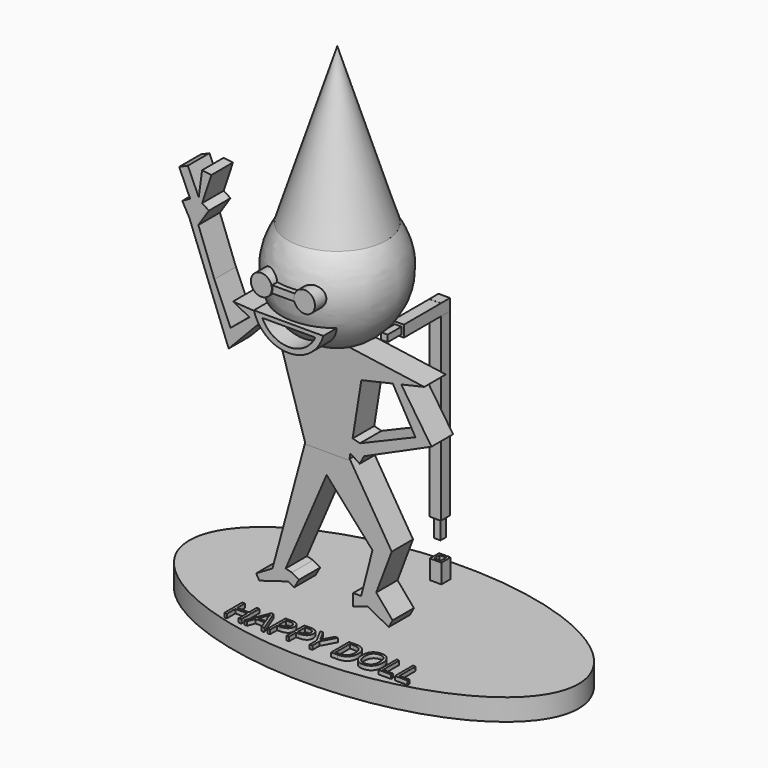
from build123d import *

# Parameters (mm, degrees)
F4_R          = 1.3944726586
F5_DEPTH      = 8.83985
F6_W          = 3.6523307208
F6_H          = 0.9525045753
F7_DEPTH      = 8.73121
F9_DEPTH      = 8.04328
F11_DEPTH     = 1.790545
F13_DEPTH     = 1.76659
F17_W         = 1.524
F17_H         = 1.524
F17_W_2       = 0.889
F17_H_2       = 0.889
F18_DEPTH     = 2.54
F21_DEPTH     = 2.87519
F23_W         = 1.524
F23_H         = 1.524
F23_W_2       = 0.889
F23_H_2       = 0.889
F24_DEPTH     = 2.54
F25_W         = 1.524
F25_H         = 1.524
F26_DEPTH     = 25.4
F28_W         = 0.889
F28_H         = 0.889
F29_DEPTH     = 2.54
F31_W         = 1.524
F31_H         = 1.524
F32_DEPTH     = 7.62
F34_W         = 0.889
F34_H         = 0.889
F35_DEPTH     = 2.286
F40_TEXT_SIZE = 4.1768032437
F41_DEPTH     = 0.52886


# Not quite as in the source:
# - a feature names something its author has since deleted; it is built from what else it names
# - Text() gives the source's letters only with a copy of the font that has no kerning and outlines rounded to 1/6400 em; it was checked with that copy


with BuildPart() as f1:
    # F0 (on Front) → F1 (revolve)
    with BuildSketch(Plane.XZ):
        with BuildLine():
            Line((0, 41.7647510767), (0, 24.1672452539))
            ThreePointArc((0, 24.1672452539), (8.0870628543, 32.9659981653), (0, 41.7647510767))
        make_face()
    revolve(axis=Axis((0, 0, 32.9659981653), (0, 0, 1)))

    # F4 (on Front) → F5 (join)
    with BuildSketch(Plane.XZ):
        with Locations((2.7146725915, 33.2950428128)):
            Circle(F4_R)
        with Locations((-3.0039404519, 33.4141813219)):
            Circle(F4_R)
    extrude(amount=F5_DEPTH)

    # F6 (on Front) → F7 (join)
    with BuildSketch(Plane.XZ):
        with Locations((0, 33.295340836)):
            Rectangle(F6_W, F6_H)
    extrude(amount=F7_DEPTH)

    # F8 (on Front) → F9 (join)
    with BuildSketch(Plane.XZ):
        with BuildLine():
            Line((4.5767659321, 29.5911673456), (-4.6307551675, 29.5911673456))
            ThreePointArc((-4.6307551675, 29.5911673456), (-0.0269946177, 26.1003461739), (4.5767659321, 29.5911673456))
        make_face()
        with BuildLine():
            ThreePointArc((3.5184309818, 29.061999172), (-0.0005357433, 26.8033396538), (-3.5195024684, 29.061999172))
            Line((-3.5195024684, 29.061999172), (3.5184309818, 29.061999172))
        make_face(mode=Mode.SUBTRACT)
    extrude(amount=F9_DEPTH)


with BuildPart() as f3:
    # F2 (on Front) → F3 (revolve)
    with BuildSketch(Plane.XZ):
        with BuildLine():
            Line((0, 58.7905235589), (0, 41.872959584))
            add(Edge.make_bspline(
                [(0, 41.872959584), (1.0115341242, 41.5872805724), (2.9001635697, 41.0538909612), (4.6529319552, 39.7735674728), (6.1744177712, 38.7379163375), (6.5332196187, 38.2138098642)],
                knots=[0, 0, 0, 0, 0.2961865012, 0.5530080837, 0.8154471343, 0.8154471343, 0.8154471343, 0.8154471343], degree=3))
            Line((6.5332196187, 38.2138098642), (0, 58.7905235589))
        make_face()
    revolve(axis=Axis((0, 0, 50.3317415714), (0, 0, 1)))


with BuildPart() as f11:
    # F10 (on Front) → F11 (new body, symmetric)
    with BuildSketch(Plane.XZ):
        Polygon((-0.3933850094, 24.2639351636), (-1.3308248017, 24.4045499712), (-12.3926112428, 25.1545030624), (-10.2172776953, 24.0195461021), (-9.1584448237, 23.4671114013), (-5.9242784046, 21.7797197402), (-2.783855889, 11.6085018963), (3.0282693915, 11.6085018963), (3.1673764521, 12.4717842192), (3.0165510252, 12.5693771988), (3.4639604713, 14.3123503261), (4.6219159849, 21.4984882623), (8.7935219053, 22.4593635648), (9.9121591737, 22.7170271467), (12.9651278257, 23.4202388674), (2.7001653798, 24.8732697219), (1.1533898069, 24.2639351636), align=None)
        Polygon((-9.1584448237, 23.4671114013), (-10.2172776953, 24.0195461021), (-12.7207143232, 21.9672080129), (-14.876825735, 26.9356369972), (-16.9977825135, 32.5837098062), (-15.6033411622, 34.716386348), (-16.4961919175, 35.3001729604), (-15.2752371505, 38.9817357063), (-16.5056269616, 39.1457863152), (-16.9483485411, 35.8253468223), (-18.3922238648, 39.0637628734), (-19.5406130612, 38.5517437886), (-18.0894707231, 35.2970288124), (-19.1304571927, 34.716386348), (-18.1875725122, 33.0259653835), (-12.9785109311, 19.4595567882), align=None)
        Polygon((13.9260031283, 16.7527012527), (9.9121591737, 22.7170271467), (8.7935219053, 22.4593635648), (11.7933275178, 17.1628296375), (4.4343227919, 14.0632648631), (3.4639604713, 14.3123503261), (3.1673764521, 12.4717842192), (4.4109919108, 11.6670913994), (4.9851736985, 12.733428739), align=None)
        Polygon((3.0165510252, 12.5693771988), (3.1673764521, 12.4717842192), (3.4639604713, 14.3123503261), align=None)
    extrude(amount=F11_DEPTH, both=True)


with BuildPart() as f13:
    # F12 (on Front) → F13 (new body, symmetric)
    with BuildSketch(Plane.XZ):
        Polygon((2.9717034195, 11.635068804), (-2.8557472397, 11.4685697481), (-7.1847108193, -4.626294598), (-9.3491924927, -5.9027834795), (-8.9276397039, -6.6175905561), (-5.0757285208, -5.4587870836), (-4.29873541, -5.9027834795), (-3.6771403554, -4.8149929489), (-4.6214864438, -4.2753662085), (-5.4346419236, -4.0566554209), (0, 8.6380941793), (6.0796770267, 1.8116513966), (4.5811892487, -4.0157996118), (3.5266987979, -4.0157996118), (3.5266987979, -5.569786299), (5.4136822, -4.9592913128), (8.2441587001, -6.4577790909), (8.7450046825, -5.511736818), (6.5791727975, -2.9613084625), (8.6326552555, 2.4776456412), align=None)
    extrude(amount=F13_DEPTH, both=True)


with BuildPart() as f13_1:
    # F14: moved
    add(f13.part.moved(Location((0, 0, 0.28837))))


with BuildPart() as f1_1:
    # F15: moved
    add(f1.part.moved(Location((0, 0, -0.40026))))


with BuildPart() as f3_1:
    # F16: moved
    add(f3.part.moved(Location((0, 0, -0.5109))))


with BuildPart() as f18:
    # F17 (on Front) → F18 (new body)
    with BuildSketch(Plane.XZ):
        with Locations((0, 12.9114145067)):
            Rectangle(F17_W, F17_H)
        with Locations((0, 12.9114145067)):
            Rectangle(F17_W_2, F17_H_2, mode=Mode.SUBTRACT)
    extrude(amount=-F18_DEPTH)


with BuildPart() as f18_1:
    # F19: moved
    add(f18.part.moved(Location((0, 0, 7.06322))))


with BuildPart() as f21:
    # F20 (on Top) → F21 (new body)
    with BuildSketch(Plane.XY):
        with BuildLine():
            add(Edge.make_bspline(
                [(25.8096773177, 28.6252778023), (25.8096773177, 51.3844503494), (-12.9048386589, 40.0048640759), (-51.6193546355, 28.6252778023), (-12.9048386589, 17.2456915288), (25.8096773177, 5.8661052552), (25.8096773177, 28.6252778023)],
                knots=[0, 0, 0, 2.0943951024, 2.0943951024, 4.1887902048, 4.1887902048, 6.2831853072, 6.2831853072, 6.2831853072], degree=2, weights=[1, 0.5, 1, 0.5, 1, 0.5, 1]))
        make_face()
    extrude(amount=F21_DEPTH)


with BuildPart() as f21_1:
    # F22: moved
    add(f21.part.moved(Location((0, 0, -20.17848))))

    # F40 (on face) → F41 (join)
    with BuildSketch(Plane.XY.offset(-17.30329)):
        with Locations((-12.5886274036, 17.3646416515)):
            Text('HAPPY DOLL', F40_TEXT_SIZE, font='Open Sans', text_align=(TextAlign.LEFT, TextAlign.BOTTOM))
    extrude(amount=F41_DEPTH)


with BuildPart() as f24:
    # F23 (on face) → F24 (new body)
    with BuildSketch(Plane.XY.offset(-17.30329)):
        with Locations((0, 37.9488207861)):
            Rectangle(F23_W, F23_H)
        with Locations((0, 37.9488207861)):
            Rectangle(F23_W_2, F23_H_2, mode=Mode.SUBTRACT)
    extrude(amount=F24_DEPTH)


with BuildPart() as f26:
    # F25 (on Top) → F26 (new body)
    with BuildSketch(Plane.XY):
        with Locations((0, 22.6533336764)):
            Rectangle(F25_W, F25_H)
    extrude(amount=F26_DEPTH)


with BuildPart() as f26_1:
    # F27: moved
    add(f26.part.moved(Location((0, 15.20225, -9.83139))))


with BuildPart() as f29:
    # F28 (on face) → F29 (new body)
    with BuildSketch(Plane(origin=(0, 0, -9.83139), x_dir=(1, 0, 0), z_dir=(0, 0, -1))):
        with Locations((0, -32.6515906835)):
            Rectangle(F28_W, F28_H)
    extrude(amount=F29_DEPTH)


with BuildPart() as f29_1:
    # F30: moved
    add(f29.part.moved(Location((0, 5.23007, 0))))


with BuildPart() as f32:
    # F31 (on face) → F32 (new body)
    with BuildSketch(Plane(origin=(0, 2.54, 0), x_dir=(-1, 0, 0), z_dir=(0, 1, 0))):
        with Locations((0, 27.1528068134)):
            Rectangle(F31_W, F31_H)
    extrude(amount=F32_DEPTH)


with BuildPart() as f32_1:
    # F33: moved
    add(f32.part.moved(Location((0, 28.43152, -12.35574))))


with BuildPart() as f35:
    # F34 (on face) → F35 (new body)
    with BuildSketch(Plane.XZ.offset(-30.97152)):
        with Locations((0, 26.2114275247)):
            Rectangle(F34_W, F34_H)
    extrude(amount=F35_DEPTH)


with BuildPart() as f1_2:
    # F36: moved
    add(f1_1.part.moved(Location((0, 20.88237, -6.3351))))


with BuildPart() as f3_2:
    # F36: moved
    add(f3_1.part.moved(Location((0, 20.88237, -6.3351))))


with BuildPart() as f11_1:
    # F36: moved
    add(f11.part.moved(Location((0, 20.88237, -6.3351))))


with BuildPart() as f13_2:
    # F36: moved
    add(f13_1.part.moved(Location((0, 20.88237, -6.3351))))


with BuildPart() as f18_2:
    # F36: moved
    add(f18_1.part.moved(Location((0, 20.88237, -6.3351))))


with BuildPart() as f35_1:
    # F37: moved
    add(f35.part.moved(Location((0, 0, -11.43434))))


with BuildPart() as f18_3:
    # F38: moved
    add(f18_2.part.moved(Location((0, 1.82534, 0))))


with BuildPart() as f18_4:
    # F39: moved
    add(f18_3.part.moved(Location((0, 0, -1.21526))))


solid = Compound([f21_1.part, f24.part, f26_1.part, f29_1.part, f32_1.part, f1_2.part, f3_2.part, f11_1.part, f13_2.part, f35_1.part, f18_4.part])
